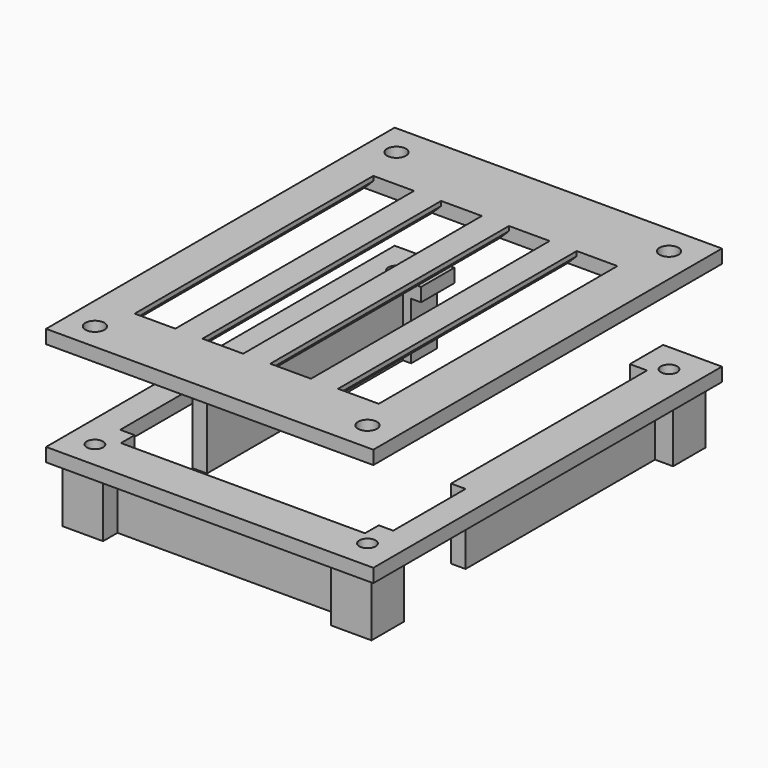
from build123d import *

# Parameters (mm, degrees)
F0_W     = 1.6
F0_H     = 1
F1_DEPTH = 7.8
F0_H_2   = 26.2
F0_W_2   = 0.5
F2_DEPTH = 1.5
F3_DEPTH = 7.8
F5_R     = 0.9
F6_DEPTH = 8
F8_R     = 1.05
F8_W     = 4.5
F8_H     = 33
F9_DEPTH = 1.5
F10_SIZE = 1


# Not quite as in the source:
# - a feature names something its author has since deleted; it is built from what else it names


with BuildPart() as f1:
    # F0 (on Top) → F1 (new body)
    with BuildSketch(Plane.XY):
        with BuildLine():
            Line((-14.1721238852, -28.8496168345), (-14.1721238852, -27.9496168345))
            Line((-14.1721238852, -27.9496168345), (-15.7721238852, -27.9496168345))
            Line((-15.7721238852, -27.9496168345), (-15.7721238852, -28.4496168345))
            ThreePointArc((-15.7721238852, -28.4496168345), (-14.3579103228, -29.0354032721), (-13.7721238852, -30.4496168345))
            Line((-13.7721238852, -30.4496168345), (-13.2721238852, -30.4496168345))
            Line((-13.2721238852, -30.4496168345), (-13.2721238852, -28.8496168345))
            Line((-13.2721238852, -28.8496168345), (-14.1721238852, -28.8496168345))
        make_face()
        Polygon((11.9278761148, -28.8496168345), (-13.2721238852, -28.8496168345), (-13.2721238852, -30.4496168345), (11.9278761148, -30.4496168345), (11.9278761148, -30.1996168345), align=None)
        with BuildLine():
            Line((12.3778761148, -28.8496168345), (11.9278761148, -28.8496168345))
            Line((11.9278761148, -28.8496168345), (11.9278761148, -30.1996168345))
            ThreePointArc((11.9278761148, -30.1996168345), (12.0433386942, -29.488104361), (12.3778761148, -28.8496168345))
        make_face()
        with BuildLine():
            ThreePointArc((14.1778761148, -27.9496168345), (13.4663636413, -28.0650794139), (12.8278761148, -28.3996168345))
            Line((12.8278761148, -28.3996168345), (12.8278761148, -28.8496168345))
            Line((12.8278761148, -28.8496168345), (12.3778761148, -28.8496168345))
            ThreePointArc((12.3778761148, -28.8496168345), (12.0433386942, -29.488104361), (11.9278761148, -30.1996168345))
            ThreePointArc((11.9278761148, -30.1996168345), (11.9313618205, -30.3248107853), (11.9418081373, -30.4496168345))
            Line((11.9418081373, -30.4496168345), (14.4278761148, -30.4496168345))
            Line((14.4278761148, -30.4496168345), (14.4278761148, -27.963548857))
            ThreePointArc((14.4278761148, -27.963548857), (14.3030700656, -27.9531025402), (14.1778761148, -27.9496168345))
        make_face()
        with BuildLine():
            Line((14.1778761148, -27.9496168345), (12.8278761148, -27.9496168345))
            Line((12.8278761148, -27.9496168345), (12.8278761148, -28.3996168345))
            ThreePointArc((12.8278761148, -28.3996168345), (13.4663636413, -28.0650794139), (14.1778761148, -27.9496168345))
        make_face()
        with BuildLine():
            ThreePointArc((11.9418081373, -30.4496168345), (11.9313618205, -30.3248107853), (11.9278761148, -30.1996168345))
            Line((11.9278761148, -30.1996168345), (11.9278761148, -30.4496168345))
            Line((11.9278761148, -30.4496168345), (11.9418081373, -30.4496168345))
        make_face()
        with BuildLine():
            Line((14.4278761148, -27.9496168345), (14.1778761148, -27.9496168345))
            ThreePointArc((14.1778761148, -27.9496168345), (14.3030700656, -27.9531025402), (14.4278761148, -27.963548857))
            Line((14.4278761148, -27.963548857), (14.4278761148, -27.9496168345))
        make_face()
        with BuildLine():
            ThreePointArc((-13.7721238852, -30.4496168345), (-14.3579103228, -29.0354032721), (-15.7721238852, -28.4496168345))
            Line((-15.7721238852, -28.4496168345), (-15.7721238852, -30.4496168345))
            Line((-15.7721238852, -30.4496168345), (-13.7721238852, -30.4496168345))
        make_face()
        with Locations((-14.9721238852, -27.4496168345)):
            Rectangle(F0_W, F0_H)
        Polygon((14.4278761148, -26.9496168345), (12.8278761148, -26.9496168345), (12.8278761148, -27.9496168345), (14.1778761148, -27.9496168345), (14.4278761148, -27.9496168345), align=None)
    extrude(amount=-F1_DEPTH)



with BuildPart() as f1b:
    # F0 (on Top) → F1, piece 2 (new body)
    with BuildSketch(Plane.XY):
        Polygon((14.1778761148, 9.2503831655), (12.8278761148, 9.2503831655), (12.8278761148, -16.9496168345), (14.4278761148, -16.9496168345), (14.4278761148, 9.2503831655), align=None)
        with BuildLine():
            ThreePointArc((11.9278761148, 11.5003831655), (12.0433386942, 10.7888706919), (12.3778761148, 10.1503831655))
            Line((12.3778761148, 10.1503831655), (12.8278761148, 10.1503831655))
            Line((12.8278761148, 10.1503831655), (12.8278761148, 9.7003831655))
            ThreePointArc((12.8278761148, 9.7003831655), (13.4663636413, 9.3658457449), (14.1778761148, 9.2503831655))
            ThreePointArc((14.1778761148, 9.2503831655), (14.3030700656, 9.2538688711), (14.4278761148, 9.264315188))
            Line((14.4278761148, 9.264315188), (14.4278761148, 11.7503831655))
            Line((14.4278761148, 11.7503831655), (11.9418081373, 11.7503831655))
            ThreePointArc((11.9418081373, 11.7503831655), (11.9313618205, 11.6255771163), (11.9278761148, 11.5003831655))
        make_face()
        with BuildLine():
            Line((11.9278761148, 11.5003831655), (11.9278761148, 10.1503831655))
            Line((11.9278761148, 10.1503831655), (12.3778761148, 10.1503831655))
            ThreePointArc((12.3778761148, 10.1503831655), (12.0433386942, 10.7888706919), (11.9278761148, 11.5003831655))
        make_face()
        with BuildLine():
            Line((11.9278761148, 11.7503831655), (11.9278761148, 11.5003831655))
            ThreePointArc((11.9278761148, 11.5003831655), (11.9313618205, 11.6255771163), (11.9418081373, 11.7503831655))
            Line((11.9418081373, 11.7503831655), (11.9278761148, 11.7503831655))
        make_face()
        with BuildLine():
            ThreePointArc((14.4278761148, 9.264315188), (14.3030700656, 9.2538688711), (14.1778761148, 9.2503831655))
            Line((14.1778761148, 9.2503831655), (14.4278761148, 9.2503831655))
            Line((14.4278761148, 9.2503831655), (14.4278761148, 9.264315188))
        make_face()
        with BuildLine():
            ThreePointArc((14.1778761148, 9.2503831655), (13.4663636413, 9.3658457449), (12.8278761148, 9.7003831655))
            Line((12.8278761148, 9.7003831655), (12.8278761148, 9.2503831655))
            Line((12.8278761148, 9.2503831655), (14.1778761148, 9.2503831655))
        make_face()
    extrude(amount=-F1_DEPTH)


with BuildPart() as f1c:
    # F0 (on Top) → F1, piece 3 (new body)
    with BuildSketch(Plane.XY):
        with Locations((-14.9721238852, -3.8496168345)):
            Rectangle(F0_W, F0_H_2)
        with BuildLine():
            Line((-14.1017945763, 10.1503831655), (-13.2721238852, 10.1503831655))
            Line((-13.2721238852, 10.1503831655), (-13.2721238852, 13.7503831655))
            Line((-13.2721238852, 13.7503831655), (-13.7721238852, 13.7503831655))
            Line((-13.7721238852, 13.7503831655), (-13.7721238852, 11.7503831655))
            Line((-13.7721238852, 11.7503831655), (-13.8356322121, 11.7503831655))
            ThreePointArc((-13.8356322121, 11.7503831655), (-13.7880644926, 11.5023917504), (-13.7721238852, 11.2503831655))
            ThreePointArc((-13.7721238852, 11.2503831655), (-13.8563135321, 10.6762135989), (-14.1017945763, 10.1503831655))
        make_face()
        with BuildLine():
            Line((-14.1721238852, 9.2503831655), (-14.1721238852, 10.0503831655))
            ThreePointArc((-14.1721238852, 10.0503831655), (-14.8776966942, 9.4615287835), (-15.7721238852, 9.2503831655))
            Line((-15.7721238852, 9.2503831655), (-14.1721238852, 9.2503831655))
        make_face()
        with BuildLine():
            Line((-14.1721238852, 10.1503831655), (-14.1017945763, 10.1503831655))
            ThreePointArc((-14.1017945763, 10.1503831655), (-13.8563135321, 10.6762135989), (-13.7721238852, 11.2503831655))
            ThreePointArc((-13.7721238852, 11.2503831655), (-13.7880644926, 11.5023917504), (-13.8356322121, 11.7503831655))
            Line((-13.8356322121, 11.7503831655), (-15.7721238852, 11.7503831655))
            Line((-15.7721238852, 11.7503831655), (-15.7721238852, 9.2503831655))
            ThreePointArc((-15.7721238852, 9.2503831655), (-14.8776966942, 9.4615287835), (-14.1721238852, 10.0503831655))
            Line((-14.1721238852, 10.0503831655), (-14.1721238852, 10.1503831655))
        make_face()
    extrude(amount=-F1_DEPTH)


with BuildPart() as f1_1:
    add(f1.part)

    add(f1b.part)  # F2 merges F1b

    add(f1c.part)  # F2 merges F1c
    # F0 (on Top) → F2 (join)
    with BuildSketch(Plane.XY):
        Polygon((10.9278761148, 14.7503831655), (10.9278761148, 11.7503831655), (11.9278761148, 11.7503831655), (11.9278761148, 13.7503831655), (14.177876148, 13.7503831655), (16.4278761148, 13.7503831655), (16.4278761148, 11.5003831655), (16.4278761148, 9.2503831655), (14.4278761148, 9.2503831655), (14.4278761148, -16.9496168345), (14.4278761148, -26.9496168345), (14.4278761148, -27.9496168345), (16.4278761148, -27.9496168345), (16.4278761148, -30.1996168345), (16.4278761148, -32.4496168345), (14.1778761148, -32.4496168345), (11.9278761148, -32.4496168345), (11.9278761148, -30.4496168345), (-13.2721238852, -30.4496168345), (-13.2721238852, -32.4496168345), (-15.7721238852, -32.4496168345), (-17.7721238852, -32.4496168345), (-17.7721238852, -30.4496168345), (-17.7721238852, -27.9496168345), (-15.7721238852, -27.9496168345), (-15.7721238852, -26.9496168345), (-15.7721238852, -16.9496168345), (-15.7721238852, 9.2503831655), (-17.7721238852, 9.2503831655), (-17.7721238852, 11.2503831655), (-17.7721238852, 13.7503831655), (-13.7721238852, 13.7503831655), (-13.7721238852, 14.7503831655), (-18.7721238852, 14.7503831655), (-18.7721238852, -33.4496168345), (17.4278761148, -33.4496168345), (17.4278761148, 14.7503831655), align=None)
        with BuildLine():
            Line((-13.7721238852, 11.7503831655), (-13.7721238852, 13.7503831655))
            Line((-13.7721238852, 13.7503831655), (-17.7721238852, 13.7503831655))
            Line((-17.7721238852, 13.7503831655), (-17.7721238852, 11.2503831655))
            ThreePointArc((-17.7721238852, 11.2503831655), (-16.0241324701, 13.234442558), (-13.8356322121, 11.7503831655))
            Line((-13.8356322121, 11.7503831655), (-13.7721238852, 11.7503831655))
        make_face()
        with BuildLine():
            ThreePointArc((-17.7721238852, 11.2503831655), (-17.1863374475, 9.8361696031), (-15.7721238852, 9.2503831655))
            Line((-15.7721238852, 9.2503831655), (-15.7721238852, 11.7503831655))
            Line((-15.7721238852, 11.7503831655), (-13.8356322121, 11.7503831655))
            ThreePointArc((-13.8356322121, 11.7503831655), (-16.0241324701, 13.234442558), (-17.7721238852, 11.2503831655))
        make_face()
        with BuildLine():
            Line((-17.7721238852, 9.2503831655), (-15.7721238852, 9.2503831655))
            ThreePointArc((-15.7721238852, 9.2503831655), (-17.1863374475, 9.8361696031), (-17.7721238852, 11.2503831655))
            Line((-17.7721238852, 11.2503831655), (-17.7721238852, 9.2503831655))
        make_face()
        with BuildLine():
            Line((14.4278761148, 9.264315188), (14.4278761148, 9.2503831655))
            Line((14.4278761148, 9.2503831655), (16.4278761148, 9.2503831655))
            Line((16.4278761148, 9.2503831655), (16.4278761148, 11.5003831655))
            ThreePointArc((16.4278761148, 11.5003831655), (15.854927098, 10.0003831655), (14.4278761148, 9.264315188))
        make_face()
        with BuildLine():
            ThreePointArc((14.177876148, 13.7503831655), (12.6778761272, 13.1774341597), (11.9418081373, 11.7503831655))
            Line((11.9418081373, 11.7503831655), (14.4278761148, 11.7503831655))
            Line((14.4278761148, 11.7503831655), (14.4278761148, 9.264315188))
            ThreePointArc((14.4278761148, 9.264315188), (15.854927098, 10.0003831655), (16.4278761148, 11.5003831655))
            ThreePointArc((16.4278761148, 11.5003831655), (15.7688663842, 13.0913734114), (14.177876148, 13.7503831655))
        make_face()
        with BuildLine():
            Line((16.4278761148, 13.7503831655), (14.177876148, 13.7503831655))
            ThreePointArc((14.177876148, 13.7503831655), (15.7688663842, 13.0913734114), (16.4278761148, 11.5003831655))
            Line((16.4278761148, 11.5003831655), (16.4278761148, 13.7503831655))
        make_face()
        with BuildLine():
            Line((11.9278761148, 13.7503831655), (11.9278761148, 11.7503831655))
            Line((11.9278761148, 11.7503831655), (11.9418081373, 11.7503831655))
            ThreePointArc((11.9418081373, 11.7503831655), (12.6778761272, 13.1774341597), (14.177876148, 13.7503831655))
            Line((14.177876148, 13.7503831655), (11.9278761148, 13.7503831655))
        make_face()
        with BuildLine():
            Line((-13.2721238852, -30.4496168345), (-13.7721238852, -30.4496168345))
            ThreePointArc((-13.7721238852, -30.4496168345), (-14.3579103228, -31.8638303969), (-15.7721238852, -32.4496168345))
            Line((-15.7721238852, -32.4496168345), (-13.2721238852, -32.4496168345))
            Line((-13.2721238852, -32.4496168345), (-13.2721238852, -30.4496168345))
        make_face()
        with BuildLine():
            Line((-15.7721238852, -30.4496168345), (-15.7721238852, -28.4496168345))
            ThreePointArc((-15.7721238852, -28.4496168345), (-17.1863374475, -29.0354032721), (-17.7721238852, -30.4496168345))
            ThreePointArc((-17.7721238852, -30.4496168345), (-17.1863374475, -31.8638303969), (-15.7721238852, -32.4496168345))
            ThreePointArc((-15.7721238852, -32.4496168345), (-14.3579103228, -31.8638303969), (-13.7721238852, -30.4496168345))
            Line((-13.7721238852, -30.4496168345), (-15.7721238852, -30.4496168345))
        make_face()
        with BuildLine():
            ThreePointArc((-15.7721238852, -32.4496168345), (-17.1863374475, -31.8638303969), (-17.7721238852, -30.4496168345))
            Line((-17.7721238852, -30.4496168345), (-17.7721238852, -32.4496168345))
            Line((-17.7721238852, -32.4496168345), (-15.7721238852, -32.4496168345))
        make_face()
        with BuildLine():
            Line((-15.7721238852, -28.4496168345), (-15.7721238852, -27.9496168345))
            Line((-15.7721238852, -27.9496168345), (-17.7721238852, -27.9496168345))
            Line((-17.7721238852, -27.9496168345), (-17.7721238852, -30.4496168345))
            ThreePointArc((-17.7721238852, -30.4496168345), (-17.1863374475, -29.0354032721), (-15.7721238852, -28.4496168345))
        make_face()
        with BuildLine():
            Line((16.4278761148, -27.9496168345), (14.4278761148, -27.9496168345))
            Line((14.4278761148, -27.9496168345), (14.4278761148, -27.963548857))
            ThreePointArc((14.4278761148, -27.963548857), (15.854927098, -28.6996168345), (16.4278761148, -30.1996168345))
            Line((16.4278761148, -30.1996168345), (16.4278761148, -27.9496168345))
        make_face()
        with BuildLine():
            ThreePointArc((16.4278761148, -30.1996168345), (15.854927098, -28.6996168345), (14.4278761148, -27.963548857))
            Line((14.4278761148, -27.963548857), (14.4278761148, -30.4496168345))
            Line((14.4278761148, -30.4496168345), (11.9418081373, -30.4496168345))
            ThreePointArc((11.9418081373, -30.4496168345), (12.6778761148, -31.8766678176), (14.1778761148, -32.4496168345))
            ThreePointArc((14.1778761148, -32.4496168345), (15.7688663725, -31.7906070922), (16.4278761148, -30.1996168345))
        make_face()
        with BuildLine():
            Line((16.4278761148, -32.4496168345), (16.4278761148, -30.1996168345))
            ThreePointArc((16.4278761148, -30.1996168345), (15.7688663725, -31.7906070922), (14.1778761148, -32.4496168345))
            Line((14.1778761148, -32.4496168345), (16.4278761148, -32.4496168345))
        make_face()
        with BuildLine():
            Line((11.9418081373, -30.4496168345), (11.9278761148, -30.4496168345))
            Line((11.9278761148, -30.4496168345), (11.9278761148, -32.4496168345))
            Line((11.9278761148, -32.4496168345), (14.1778761148, -32.4496168345))
            ThreePointArc((14.1778761148, -32.4496168345), (12.6778761148, -31.8766678176), (11.9418081373, -30.4496168345))
        make_face()
        with Locations((-13.5221238852, 14.2503831655)):
            Rectangle(F0_W_2, F0_H)
        with BuildLine():
            Line((-14.1017945763, 10.1503831655), (-13.2721238852, 10.1503831655))
            Line((-13.2721238852, 10.1503831655), (-13.2721238852, 13.7503831655))
            Line((-13.2721238852, 13.7503831655), (-13.7721238852, 13.7503831655))
            Line((-13.7721238852, 13.7503831655), (-13.7721238852, 11.7503831655))
            Line((-13.7721238852, 11.7503831655), (-13.8356322121, 11.7503831655))
            ThreePointArc((-13.8356322121, 11.7503831655), (-13.7880644926, 11.5023917504), (-13.7721238852, 11.2503831655))
            ThreePointArc((-13.7721238852, 11.2503831655), (-13.8563135321, 10.6762135989), (-14.1017945763, 10.1503831655))
        make_face()
        Polygon((-13.2721238852, 10.1503831655), (-12.1721238852, 10.1503831655), (-12.1721238852, 14.7503831655), (-13.2721238852, 14.7503831655), (-13.2721238852, 13.7503831655), align=None)
        Polygon((10.9278761148, 11.7503831655), (10.9278761148, 10.1503831655), (11.9278761148, 10.1503831655), (11.9278761148, 11.5003831655), (11.9278761148, 11.7503831655), align=None)
    extrude(amount=-F2_DEPTH)

    # F0 (on Top) → F3 (join)
    with BuildSketch(Plane.XY):
        with BuildLine():
            ThreePointArc((14.177876148, 13.7503831655), (12.6778761272, 13.1774341597), (11.9418081373, 11.7503831655))
            Line((11.9418081373, 11.7503831655), (14.4278761148, 11.7503831655))
            Line((14.4278761148, 11.7503831655), (14.4278761148, 9.264315188))
            ThreePointArc((14.4278761148, 9.264315188), (15.854927098, 10.0003831655), (16.4278761148, 11.5003831655))
            ThreePointArc((16.4278761148, 11.5003831655), (15.7688663842, 13.0913734114), (14.177876148, 13.7503831655))
        make_face()
        with BuildLine():
            ThreePointArc((14.1778761148, 9.2503831655), (13.4663636413, 9.3658457449), (12.8278761148, 9.7003831655))
            Line((12.8278761148, 9.7003831655), (12.8278761148, 9.2503831655))
            Line((12.8278761148, 9.2503831655), (14.1778761148, 9.2503831655))
        make_face()
        with BuildLine():
            Line((11.9278761148, 13.7503831655), (11.9278761148, 11.7503831655))
            Line((11.9278761148, 11.7503831655), (11.9418081373, 11.7503831655))
            ThreePointArc((11.9418081373, 11.7503831655), (12.6778761272, 13.1774341597), (14.177876148, 13.7503831655))
            Line((14.177876148, 13.7503831655), (11.9278761148, 13.7503831655))
        make_face()
        with BuildLine():
            ThreePointArc((11.9278761148, 11.5003831655), (12.0433386942, 10.7888706919), (12.3778761148, 10.1503831655))
            Line((12.3778761148, 10.1503831655), (12.8278761148, 10.1503831655))
            Line((12.8278761148, 10.1503831655), (12.8278761148, 9.7003831655))
            ThreePointArc((12.8278761148, 9.7003831655), (13.4663636413, 9.3658457449), (14.1778761148, 9.2503831655))
            ThreePointArc((14.1778761148, 9.2503831655), (14.3030700656, 9.2538688711), (14.4278761148, 9.264315188))
            Line((14.4278761148, 9.264315188), (14.4278761148, 11.7503831655))
            Line((14.4278761148, 11.7503831655), (11.9418081373, 11.7503831655))
            ThreePointArc((11.9418081373, 11.7503831655), (11.9313618205, 11.6255771163), (11.9278761148, 11.5003831655))
        make_face()
        with BuildLine():
            Line((11.9278761148, 11.5003831655), (11.9278761148, 10.1503831655))
            Line((11.9278761148, 10.1503831655), (12.3778761148, 10.1503831655))
            ThreePointArc((12.3778761148, 10.1503831655), (12.0433386942, 10.7888706919), (11.9278761148, 11.5003831655))
        make_face()
        with BuildLine():
            Line((-14.1721238852, 10.1503831655), (-14.1017945763, 10.1503831655))
            ThreePointArc((-14.1017945763, 10.1503831655), (-13.8563135321, 10.6762135989), (-13.7721238852, 11.2503831655))
            ThreePointArc((-13.7721238852, 11.2503831655), (-13.7880644926, 11.5023917504), (-13.8356322121, 11.7503831655))
            Line((-13.8356322121, 11.7503831655), (-15.7721238852, 11.7503831655))
            Line((-15.7721238852, 11.7503831655), (-15.7721238852, 9.2503831655))
            ThreePointArc((-15.7721238852, 9.2503831655), (-14.8776966942, 9.4615287835), (-14.1721238852, 10.0503831655))
            Line((-14.1721238852, 10.0503831655), (-14.1721238852, 10.1503831655))
        make_face()
        with BuildLine():
            ThreePointArc((-17.7721238852, 11.2503831655), (-17.1863374475, 9.8361696031), (-15.7721238852, 9.2503831655))
            Line((-15.7721238852, 9.2503831655), (-15.7721238852, 11.7503831655))
            Line((-15.7721238852, 11.7503831655), (-13.8356322121, 11.7503831655))
            ThreePointArc((-13.8356322121, 11.7503831655), (-16.0241324701, 13.234442558), (-17.7721238852, 11.2503831655))
        make_face()
        with BuildLine():
            Line((-13.7721238852, 11.7503831655), (-13.7721238852, 13.7503831655))
            Line((-13.7721238852, 13.7503831655), (-17.7721238852, 13.7503831655))
            Line((-17.7721238852, 13.7503831655), (-17.7721238852, 11.2503831655))
            ThreePointArc((-17.7721238852, 11.2503831655), (-16.0241324701, 13.234442558), (-13.8356322121, 11.7503831655))
            Line((-13.8356322121, 11.7503831655), (-13.7721238852, 11.7503831655))
        make_face()
        with BuildLine():
            Line((-17.7721238852, 9.2503831655), (-15.7721238852, 9.2503831655))
            ThreePointArc((-15.7721238852, 9.2503831655), (-17.1863374475, 9.8361696031), (-17.7721238852, 11.2503831655))
            Line((-17.7721238852, 11.2503831655), (-17.7721238852, 9.2503831655))
        make_face()
        with BuildLine():
            Line((-14.1721238852, 9.2503831655), (-14.1721238852, 10.0503831655))
            ThreePointArc((-14.1721238852, 10.0503831655), (-14.8776966942, 9.4615287835), (-15.7721238852, 9.2503831655))
            Line((-15.7721238852, 9.2503831655), (-14.1721238852, 9.2503831655))
        make_face()
        with BuildLine():
            Line((-14.1017945763, 10.1503831655), (-13.2721238852, 10.1503831655))
            Line((-13.2721238852, 10.1503831655), (-13.2721238852, 13.7503831655))
            Line((-13.2721238852, 13.7503831655), (-13.7721238852, 13.7503831655))
            Line((-13.7721238852, 13.7503831655), (-13.7721238852, 11.7503831655))
            Line((-13.7721238852, 11.7503831655), (-13.8356322121, 11.7503831655))
            ThreePointArc((-13.8356322121, 11.7503831655), (-13.7880644926, 11.5023917504), (-13.7721238852, 11.2503831655))
            ThreePointArc((-13.7721238852, 11.2503831655), (-13.8563135321, 10.6762135989), (-14.1017945763, 10.1503831655))
        make_face()
        with BuildLine():
            Line((16.4278761148, 13.7503831655), (14.177876148, 13.7503831655))
            ThreePointArc((14.177876148, 13.7503831655), (15.7688663842, 13.0913734114), (16.4278761148, 11.5003831655))
            Line((16.4278761148, 11.5003831655), (16.4278761148, 13.7503831655))
        make_face()
        with BuildLine():
            Line((14.4278761148, 9.264315188), (14.4278761148, 9.2503831655))
            Line((14.4278761148, 9.2503831655), (16.4278761148, 9.2503831655))
            Line((16.4278761148, 9.2503831655), (16.4278761148, 11.5003831655))
            ThreePointArc((16.4278761148, 11.5003831655), (15.854927098, 10.0003831655), (14.4278761148, 9.264315188))
        make_face()
        with BuildLine():
            ThreePointArc((16.4278761148, -30.1996168345), (15.854927098, -28.6996168345), (14.4278761148, -27.963548857))
            Line((14.4278761148, -27.963548857), (14.4278761148, -30.4496168345))
            Line((14.4278761148, -30.4496168345), (11.9418081373, -30.4496168345))
            ThreePointArc((11.9418081373, -30.4496168345), (12.6778761148, -31.8766678176), (14.1778761148, -32.4496168345))
            ThreePointArc((14.1778761148, -32.4496168345), (15.7688663725, -31.7906070922), (16.4278761148, -30.1996168345))
        make_face()
        with BuildLine():
            Line((16.4278761148, -27.9496168345), (14.4278761148, -27.9496168345))
            Line((14.4278761148, -27.9496168345), (14.4278761148, -27.963548857))
            ThreePointArc((14.4278761148, -27.963548857), (15.854927098, -28.6996168345), (16.4278761148, -30.1996168345))
            Line((16.4278761148, -30.1996168345), (16.4278761148, -27.9496168345))
        make_face()
        with BuildLine():
            Line((16.4278761148, -32.4496168345), (16.4278761148, -30.1996168345))
            ThreePointArc((16.4278761148, -30.1996168345), (15.7688663725, -31.7906070922), (14.1778761148, -32.4496168345))
            Line((14.1778761148, -32.4496168345), (16.4278761148, -32.4496168345))
        make_face()
        with BuildLine():
            Line((11.9418081373, -30.4496168345), (11.9278761148, -30.4496168345))
            Line((11.9278761148, -30.4496168345), (11.9278761148, -32.4496168345))
            Line((11.9278761148, -32.4496168345), (14.1778761148, -32.4496168345))
            ThreePointArc((14.1778761148, -32.4496168345), (12.6778761148, -31.8766678176), (11.9418081373, -30.4496168345))
        make_face()
        with BuildLine():
            ThreePointArc((14.1778761148, -27.9496168345), (13.4663636413, -28.0650794139), (12.8278761148, -28.3996168345))
            Line((12.8278761148, -28.3996168345), (12.8278761148, -28.8496168345))
            Line((12.8278761148, -28.8496168345), (12.3778761148, -28.8496168345))
            ThreePointArc((12.3778761148, -28.8496168345), (12.0433386942, -29.488104361), (11.9278761148, -30.1996168345))
            ThreePointArc((11.9278761148, -30.1996168345), (11.9313618205, -30.3248107853), (11.9418081373, -30.4496168345))
            Line((11.9418081373, -30.4496168345), (14.4278761148, -30.4496168345))
            Line((14.4278761148, -30.4496168345), (14.4278761148, -27.963548857))
            ThreePointArc((14.4278761148, -27.963548857), (14.3030700656, -27.9531025402), (14.1778761148, -27.9496168345))
        make_face()
        with BuildLine():
            Line((12.3778761148, -28.8496168345), (11.9278761148, -28.8496168345))
            Line((11.9278761148, -28.8496168345), (11.9278761148, -30.1996168345))
            ThreePointArc((11.9278761148, -30.1996168345), (12.0433386942, -29.488104361), (12.3778761148, -28.8496168345))
        make_face()
        with BuildLine():
            Line((14.1778761148, -27.9496168345), (12.8278761148, -27.9496168345))
            Line((12.8278761148, -27.9496168345), (12.8278761148, -28.3996168345))
            ThreePointArc((12.8278761148, -28.3996168345), (13.4663636413, -28.0650794139), (14.1778761148, -27.9496168345))
        make_face()
        with BuildLine():
            Line((-15.7721238852, -28.4496168345), (-15.7721238852, -27.9496168345))
            Line((-15.7721238852, -27.9496168345), (-17.7721238852, -27.9496168345))
            Line((-17.7721238852, -27.9496168345), (-17.7721238852, -30.4496168345))
            ThreePointArc((-17.7721238852, -30.4496168345), (-17.1863374475, -29.0354032721), (-15.7721238852, -28.4496168345))
        make_face()
        with BuildLine():
            Line((-14.1721238852, -28.8496168345), (-14.1721238852, -27.9496168345))
            Line((-14.1721238852, -27.9496168345), (-15.7721238852, -27.9496168345))
            Line((-15.7721238852, -27.9496168345), (-15.7721238852, -28.4496168345))
            ThreePointArc((-15.7721238852, -28.4496168345), (-14.3579103228, -29.0354032721), (-13.7721238852, -30.4496168345))
            Line((-13.7721238852, -30.4496168345), (-13.2721238852, -30.4496168345))
            Line((-13.2721238852, -30.4496168345), (-13.2721238852, -28.8496168345))
            Line((-13.2721238852, -28.8496168345), (-14.1721238852, -28.8496168345))
        make_face()
        with BuildLine():
            Line((-13.2721238852, -30.4496168345), (-13.7721238852, -30.4496168345))
            ThreePointArc((-13.7721238852, -30.4496168345), (-14.3579103228, -31.8638303969), (-15.7721238852, -32.4496168345))
            Line((-15.7721238852, -32.4496168345), (-13.2721238852, -32.4496168345))
            Line((-13.2721238852, -32.4496168345), (-13.2721238852, -30.4496168345))
        make_face()
        with BuildLine():
            ThreePointArc((-15.7721238852, -32.4496168345), (-17.1863374475, -31.8638303969), (-17.7721238852, -30.4496168345))
            Line((-17.7721238852, -30.4496168345), (-17.7721238852, -32.4496168345))
            Line((-17.7721238852, -32.4496168345), (-15.7721238852, -32.4496168345))
        make_face()
        with BuildLine():
            Line((-15.7721238852, -30.4496168345), (-15.7721238852, -28.4496168345))
            ThreePointArc((-15.7721238852, -28.4496168345), (-17.1863374475, -29.0354032721), (-17.7721238852, -30.4496168345))
            ThreePointArc((-17.7721238852, -30.4496168345), (-17.1863374475, -31.8638303969), (-15.7721238852, -32.4496168345))
            ThreePointArc((-15.7721238852, -32.4496168345), (-14.3579103228, -31.8638303969), (-13.7721238852, -30.4496168345))
            Line((-13.7721238852, -30.4496168345), (-15.7721238852, -30.4496168345))
        make_face()
        with BuildLine():
            ThreePointArc((-13.7721238852, -30.4496168345), (-14.3579103228, -29.0354032721), (-15.7721238852, -28.4496168345))
            Line((-15.7721238852, -28.4496168345), (-15.7721238852, -30.4496168345))
            Line((-15.7721238852, -30.4496168345), (-13.7721238852, -30.4496168345))
        make_face()
    extrude(amount=-F3_DEPTH)

    # F5 (on offset) → F6 (cut)
    with BuildSketch(Plane.XY):
        with Locations((14.1778761148, 11.5003831655)):
            Circle(F5_R)
        with Locations((14.1778761148, -30.1996168345)):
            Circle(F5_R)
        with Locations((-15.7721238852, -30.4496168345)):
            Circle(F5_R)
        with Locations((-15.7721238852, 11.2503831655)):
            Circle(F5_R)
    extrude(amount=-F6_DEPTH, mode=Mode.SUBTRACT)


with BuildPart() as f9:
    # F8 (on offset) → F9 (new body)
    with BuildSketch(Plane.XY.offset(10)):
        Polygon((-13.7721238852, 14.7503831655), (-18.7721238852, 14.7503831655), (-18.7721238852, -33.4496168345), (17.4278761148, -33.4496168345), (17.4278761148, 14.7503831655), (10.9278761148, 14.7503831655), align=None)
        with Locations((-15.7721238852, -30.4496168345)):
            Circle(F8_R, mode=Mode.SUBTRACT)
        with Locations((-12.3221238852, -9.9496168345)):
            Rectangle(F8_W, F8_H, mode=Mode.SUBTRACT)
        with Locations((-4.8221238852, -9.9496168345)):
            Rectangle(F8_W, F8_H, mode=Mode.SUBTRACT)
        with Locations((14.1778761148, -30.1996168345)):
            Circle(F8_R, mode=Mode.SUBTRACT)
        with Locations((2.6778761148, -9.9496168345)):
            Rectangle(F8_W, F8_H, mode=Mode.SUBTRACT)
        with Locations((10.1778761148, -9.9496168345)):
            Rectangle(F8_W, F8_H, mode=Mode.SUBTRACT)
        with Locations((-15.7721238852, 11.2503831655)):
            Circle(F8_R, mode=Mode.SUBTRACT)
        with Locations((14.1778761148, 11.5003831655)):
            Circle(F8_R, mode=Mode.SUBTRACT)
    extrude(amount=F9_DEPTH)

    # F10
    f10_edges = [f9.edges().sort_by_distance(p)[0] for p in [
        (7.927876, -9.949617, 10),
        (0.427876, -9.949617, 10),
        (-7.072124, -9.949617, 10),
        (-14.572124, -9.949617, 10),
    ]]
    chamfer(f10_edges, length=F10_SIZE)


solid = Compound([f1_1.part, f9.part])
